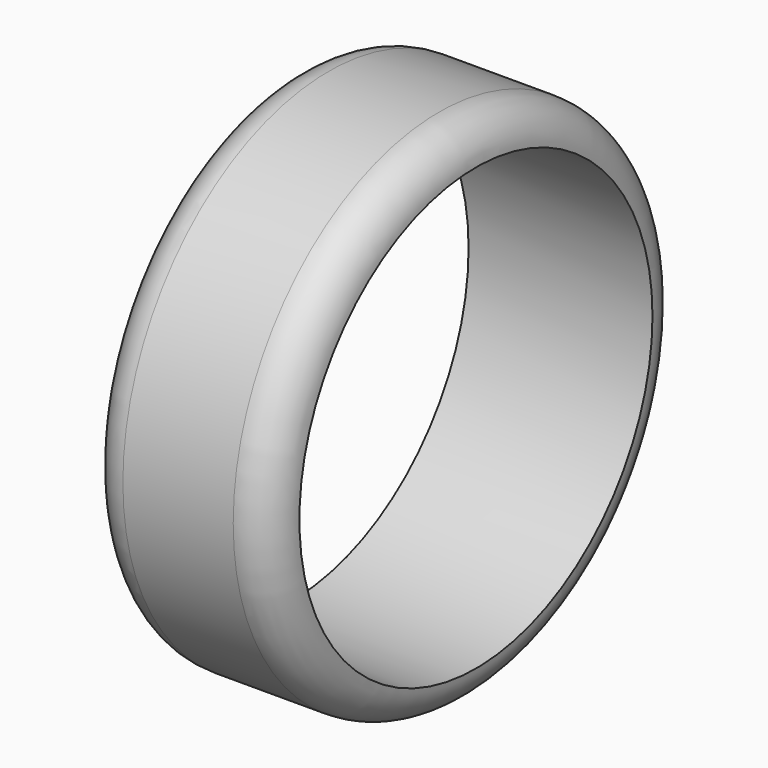
from build123d import *

# Parameters (mm, degrees)
F0_R     = 35
F0_R_2   = 30
F1_DEPTH = 25
F2_R     = 4.99999


# Not quite as in the source:
# - a fillet or chamfer is up to 0.001 mm smaller than in the source, because OpenCascade refuses the exact size


with BuildPart() as f1:
    # F0 (on Right) → F1 (new body)
    with BuildSketch(Plane.YZ):
        Circle(F0_R)
        Circle(F0_R_2, mode=Mode.SUBTRACT)
    extrude(amount=F1_DEPTH)

    # F2 (radius 5 in the source; OpenCascade refuses exactly that, so slightly less here)
    f2_edges = [f1.edges().sort_by_distance(p)[0] for p in [
        (12.5, 35, 0),
        (0, -35, 0),
        (25, -35, 0),
    ]]
    fillet(f2_edges, radius=F2_R)


solid = f1.part
